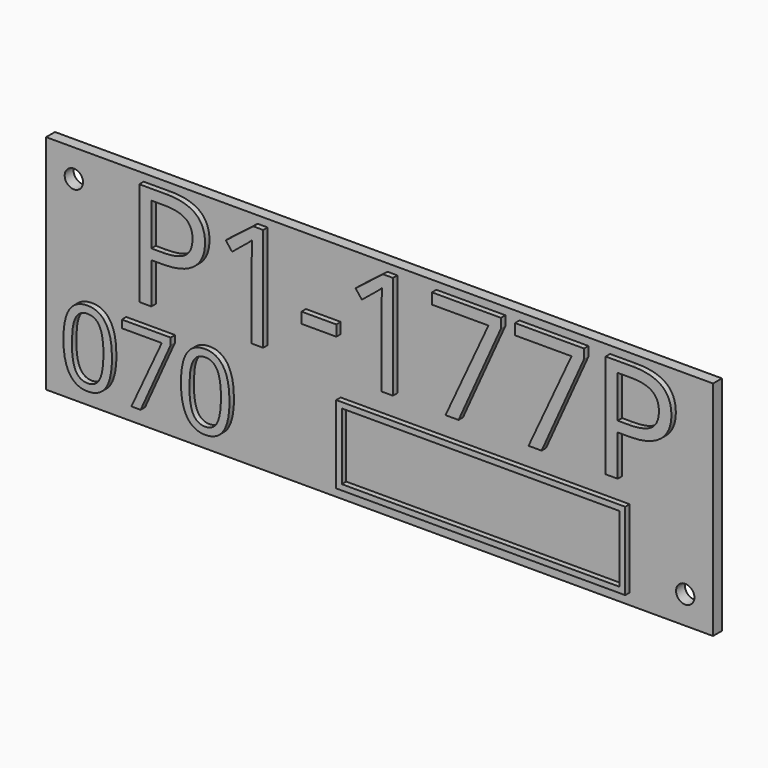
from build123d import *

# Parameters (mm, degrees)
F0_W         = 120
F0_H         = 40
F1_DEPTH     = 2
F3_D         = 3.3
F4_TEXT_SIZE = 26.1352499183
F5_DEPTH     = 1
F6_TEXT_SIZE = 18.4937691891
F7_DEPTH     = 1
F8_W         = 52
F8_H         = 14
F8_W_2       = 49.99999962
F8_H_2       = 11.99999962
F9_DEPTH     = 1


# Not quite as in the source:
# - Text() gives the source's letters only with a copy of the font that has no kerning and outlines rounded to 1/6400 em; it was checked with that copy


with BuildPart() as f1:
    # F0 (on Front) → F1 (new body)
    with BuildSketch(Plane.XZ):
        Rectangle(F0_W, F0_H)
    extrude(amount=F1_DEPTH)

    # F3 (through all)
    with Locations(Plane.XZ.offset(2)):
        with Locations((-55, 15), (55, -15)):
            Hole(F3_D / 2)

    # F4 (on face) → F5 (join)
    with BuildSketch(Plane.XZ.offset(2)):
        with Locations((-45, 0)):
            Text('P1-177P', F4_TEXT_SIZE, font='Open Sans', text_align=(TextAlign.LEFT, TextAlign.BOTTOM))
    extrude(amount=F5_DEPTH)

    # F6 (on face) → F7 (join)
    with BuildSketch(Plane.XZ.offset(2)):
        with Locations((-57, -17)):
            Text('070', F6_TEXT_SIZE, font='Open Sans', text_align=(TextAlign.LEFT, TextAlign.BOTTOM))
    extrude(amount=F7_DEPTH)

    # F8 (on face) → F9 (join)
    with BuildSketch(Plane.XZ.offset(2)):
        with Locations((19, -11)):
            Rectangle(F8_W, F8_H)
        with Locations((19, -11)):
            Rectangle(F8_W_2, F8_H_2, mode=Mode.SUBTRACT)
    extrude(amount=F9_DEPTH)


solid = f1.part
